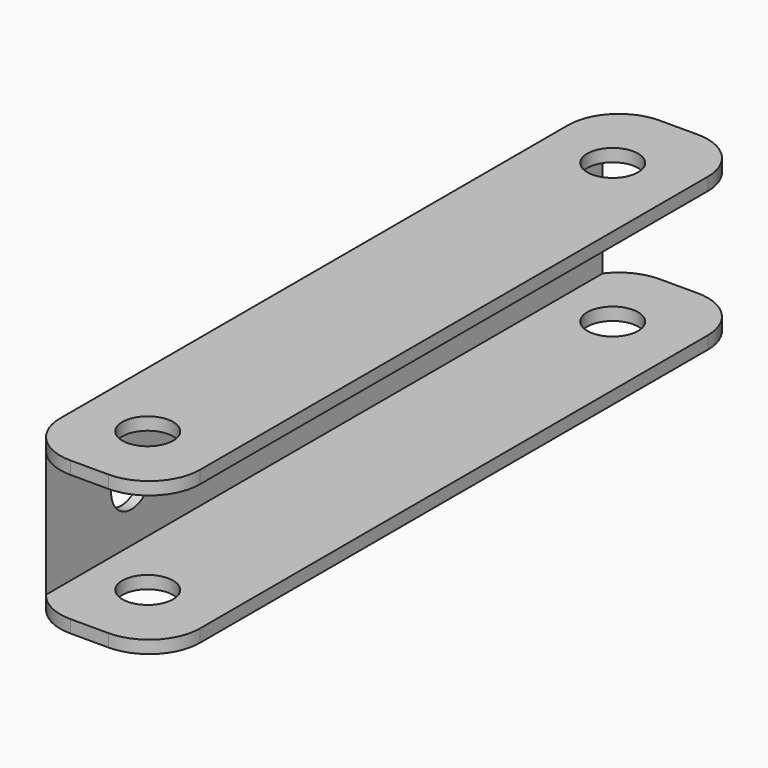
from build123d import *

# Parameters (mm, degrees)
F2_DEPTH    = 145
F1_R        = 5
F3_DEPTH    = 46
F4_T1_DEPTH = 52.5
F4_T3_DEPTH = 52.5
F4_T5_DEPTH = 80
F7_DEPTH    = 25


# Not quite as in the source:
# - a fillet or chamfer that OpenCascade refuses, or shapes differently, is made with other operations: its cross-section is extruded or revolved along the edge and cut away or added


with BuildPart() as f2:
    # F0 (on Front) → F2 (new body)
    with BuildSketch(Plane.XZ):
        Polygon((-74.9858543277, 30), (-74.9858543277, 0), (-47.4858543277, 0), (-47.4858543277, 2.5), (-72.9858543277, 2.5), (-72.9858543277, 27.5), (-47.4858543277, 27.5), (-47.4858543277, 30), align=None)
    extrude(amount=F2_DEPTH)

    # F1 (on Top) → F3 (cut)
    with BuildSketch(Plane.XY):
        with BuildLine():
            ThreePointArc((-59.9858543277, -290), (-54.9858543277, -295), (-49.9858543277, -290))
            ThreePointArc((-49.9858543277, -290), (-54.9858543277, -285), (-59.9858543277, -290))
        make_face()
        with Locations((-54.9858543277, -260)):
            Circle(F1_R)
        with Locations((-61.7693625391, -129.9988627434)):
            Circle(F1_R)
        with BuildLine():
            ThreePointArc((-61.7693625391, -20.5436318724), (-58.2338286331, -19.0791657783), (-56.7693625391, -15.5436318724))
            ThreePointArc((-56.7693625391, -15.5436318724), (-65.304896445, -12.0080979665), (-61.7693625391, -20.5436318724))
        make_face()
    extrude(amount=F3_DEPTH, mode=Mode.SUBTRACT)

    # F4: fillet of radius 10 on 6 edges, made by hand

    # F4_s2 → F4_t1 (cut)
    with BuildSketch(Plane.XY.offset(-25)):
        with BuildLine():
            ThreePointArc((-57.4858543277, 0), (-50.4147865158, -2.9289321881), (-47.4858543277, -10))
            Line((-47.4858543277, -10), (-47.4858543277, 0))
            Line((-47.4858543277, 0), (-57.4858543277, 0))
        make_face()
        with BuildLine():
            ThreePointArc((-57.4858543277, -145), (-50.4147865158, -142.0710678119), (-47.4858543277, -135))
            Line((-47.4858543277, -135), (-47.4858543277, -145))
            Line((-47.4858543277, -145), (-57.4858543277, -145))
        make_face()
    extrude(amount=F4_T1_DEPTH, mode=Mode.SUBTRACT)

    # F4_s4 → F4_t3 (cut)
    with BuildSketch(Plane.XY.offset(2.5)):
        with BuildLine():
            ThreePointArc((-47.4858543277, -10), (-50.4147865158, -2.9289321881), (-57.4858543277, 0))
            Line((-57.4858543277, 0), (-47.4858543277, 0))
            Line((-47.4858543277, 0), (-47.4858543277, -10))
        make_face()
        with BuildLine():
            ThreePointArc((-47.4858543277, -135), (-50.4147865158, -142.0710678119), (-57.4858543277, -145))
            Line((-57.4858543277, -145), (-47.4858543277, -145))
            Line((-47.4858543277, -145), (-47.4858543277, -135))
        make_face()
    extrude(amount=F4_T3_DEPTH, mode=Mode.SUBTRACT)

    # F4_s6 → F4_t5 (cut)
    with BuildSketch(Plane.XY.offset(-25)):
        with BuildLine():
            ThreePointArc((-64.9858543277, 0), (-72.0569221395, -2.9289321881), (-74.9858543277, -10))
            Line((-74.9858543277, -10), (-74.9858543277, 0))
            Line((-74.9858543277, 0), (-64.9858543277, 0))
        make_face()
        with BuildLine():
            ThreePointArc((-64.9858543277, -145), (-72.0569221395, -142.0710678119), (-74.9858543277, -135))
            Line((-74.9858543277, -135), (-74.9858543277, -145))
            Line((-74.9858543277, -145), (-64.9858543277, -145))
        make_face()
    extrude(amount=F4_T5_DEPTH, mode=Mode.SUBTRACT)

    # F6 (on offset) → F7 (cut)
    with BuildSketch(Plane(origin=(-74.9858543277, 0, 0), x_dir=(0, -1, 0), z_dir=(-1, 0, 0))):
        with BuildLine():
            ThreePointArc((30, 13.75), (21.4644660941, 17.2855339059), (25, 8.75))
            Line((25, 8.75), (25, 13.75))
            Line((25, 13.75), (30, 13.75))
        make_face()
        with BuildLine():
            Line((25, 13.75), (25, 8.75))
            ThreePointArc((25, 8.75), (28.5355339059, 10.2144660941), (30, 13.75))
            Line((30, 13.75), (25, 13.75))
        make_face()
        with BuildLine():
            Line((120, 13.75), (125, 13.75))
            ThreePointArc((125, 13.75), (120, 18.75), (115, 13.75))
            Line((115, 13.75), (120, 13.75))
        make_face()
        with BuildLine():
            ThreePointArc((115, 13.75), (120, 8.75), (125, 13.75))
            Line((125, 13.75), (120, 13.75))
            Line((120, 13.75), (115, 13.75))
        make_face()
    extrude(amount=-F7_DEPTH, mode=Mode.SUBTRACT)


solid = f2.part
